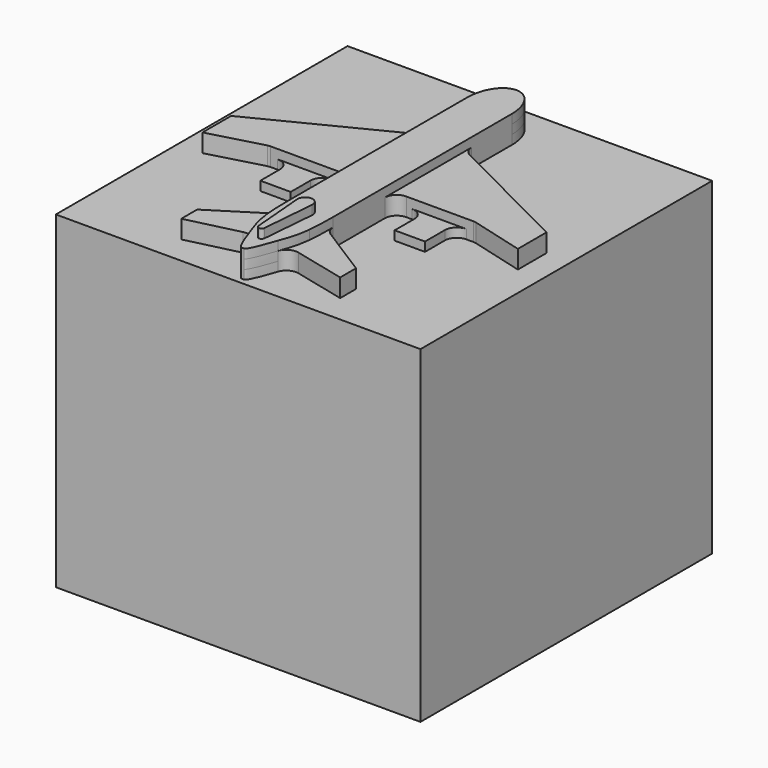
from build123d import *

# Parameters (mm, degrees)
F0_W     = 200
F0_H     = 200
F1_DEPTH = 180
F2_DEPTH = 185
F3_DEPTH = 190
F4_DEPTH = 195
F6_DEPTH = 5


with BuildPart() as f1:
    # F0 (on Top) → F1 (new body)
    with BuildSketch(Plane.XY):
        with Locations((0, -3.2757742546)):
            Rectangle(F0_W, F0_H)
        with BuildLine():
            Line((-12.2293280438, 41.5102764964), (-12.2293280438, 69.0648630261))
            add(Edge.make_bspline(
                [(12.2293280438, 69.0648630261), (12.2293280438, 87.5228339701), (0, 87.5228339701), (-12.2293280438, 87.5228339701), (-12.2293280438, 69.0648630261)],
                knots=[4.7123889804, 4.7123889804, 4.7123889804, 6.2831853072, 6.2831853072, 7.853981634, 7.853981634, 7.853981634], degree=2, weights=[1, 0.7071067812, 1, 0.7071067812, 1]))
            Line((12.2293280438, 69.0648630261), (12.2293280438, 41.5102764964))
            ThreePointArc((12.2293280438, 41.5102764964), (13.2009316357, 38.0774943136), (15.8274940025, 35.663125413))
            Line((15.8274940025, 35.663125413), (86.4709243178, 0))
            Line((86.4709243178, 0), (86.4709243178, -19.5954491359))
            Line((86.4709243178, -19.5954491359), (57.2512093193, -11.7076470548))
            ThreePointArc((57.2512093193, -11.7076470548), (56.4309868977, -11.5433023433), (55.5962785892, -11.488202028))
            Line((55.5962785892, -11.488202028), (51.7115545899, -11.488202028))
            ThreePointArc((51.7115545899, -11.488202028), (47.0800051731, -13.4066526112), (45.1615545899, -18.038202028))
            Line((45.1615545899, -18.038202028), (45.1615545899, -31.6096479073))
            Line((45.1615545899, -31.6096479073), (28.4984987229, -31.6096479073))
            Line((28.4984987229, -31.6096479073), (28.4984987229, -18.038202028))
            ThreePointArc((28.4984987229, -18.038202028), (26.5800481397, -13.4066526112), (21.9484987229, -11.488202028))
            Line((21.9484987229, -11.488202028), (18.7793280438, -11.488202028))
            ThreePointArc((18.7793280438, -11.488202028), (14.147778627, -13.4066526112), (12.2293280438, -18.038202028))
            Line((12.2293280438, -18.038202028), (12.2293280438, -53.4844789492))
            ThreePointArc((12.2293280438, -53.4844789492), (13.0425299585, -56.6454357234), (15.2802128465, -59.021508192))
            Line((15.2802128465, -59.021508192), (43.5760462728, -76.9030068116))
            Line((43.5760462728, -76.9030068116), (43.5760462728, -87.8098822028))
            Line((43.5760462728, -87.8098822028), (15.2160916988, -80.9541576008))
            ThreePointArc((15.2160916988, -80.9541576008), (10.5122070483, -81.586105591), (7.4700069214, -85.2290312635))
            add(Edge.make_bspline(
                [(7.4700069214, -85.2290312635), (4.8586251491, -93.3025441016), (1.9109145584, -100.0715989333), (0.7429708137, -100.072657045)],
                knots=[18.919621024, 18.919621024, 18.919621024, 18.919621024, 38.6142417327, 38.6142417327, 38.6142417327, 38.6142417327], degree=3))
            Line((0.7429708137, -100.072657045), (-0.7429708137, -100.072657045))
            add(Edge.make_bspline(
                [(-7.4700069214, -85.2290312635), (-4.8598522038, -93.3277695684), (-1.9207527988, -100.072657045), (-0.7429708137, -100.072657045)],
                knots=[19.243014526, 19.243014526, 19.243014526, 19.243014526, 39.0583236228, 39.0583236228, 39.0583236228, 39.0583236228], degree=3))
            ThreePointArc((-7.4700069214, -85.2290312635), (-10.5122070483, -81.586105591), (-15.2160916988, -80.9541576008))
            Line((-15.2160916988, -80.9541576008), (-43.5760462728, -87.8098822028))
            Line((-43.5760462728, -87.8098822028), (-43.5760462728, -76.9030068116))
            Line((-43.5760462728, -76.9030068116), (-15.2802128465, -59.021508192))
            ThreePointArc((-15.2802128465, -59.021508192), (-13.0425299585, -56.6454357234), (-12.2293280438, -53.4844789492))
            Line((-12.2293280438, -53.4844789492), (-12.2293280438, -18.038202028))
            ThreePointArc((-12.2293280438, -18.038202028), (-14.147778627, -13.4066526112), (-18.7793280438, -11.488202028))
            Line((-18.7793280438, -11.488202028), (-21.9484987229, -11.488202028))
            ThreePointArc((-21.9484987229, -11.488202028), (-26.5800481397, -13.4066526112), (-28.4984987229, -18.038202028))
            Line((-28.4984987229, -18.038202028), (-28.4984987229, -31.6096479073))
            Line((-28.4984987229, -31.6096479073), (-45.1615545899, -31.6096479073))
            Line((-45.1615545899, -31.6096479073), (-45.1615545899, -18.038202028))
            ThreePointArc((-45.1615545899, -18.038202028), (-47.0800051731, -13.4066526112), (-51.7115545899, -11.488202028))
            Line((-51.7115545899, -11.488202028), (-55.5962785892, -11.488202028))
            ThreePointArc((-55.5962785892, -11.488202028), (-56.4309868977, -11.5433023433), (-57.2512093193, -11.7076470548))
            Line((-57.2512093193, -11.7076470548), (-86.4709243178, -19.5954491359))
            Line((-86.4709243178, -19.5954491359), (-86.4709243178, 0))
            Line((-86.4709243178, 0), (-15.8274940025, 35.663125413))
            ThreePointArc((-15.8274940025, 35.663125413), (-13.2009316357, 38.0774943136), (-12.2293280438, 41.5102764964))
        make_face(mode=Mode.SUBTRACT)
        with BuildLine():
            add(Edge.make_bspline(
                [(12.2293280438, 69.0648630261), (12.2293280438, 87.5228339701), (0, 87.5228339701), (-12.2293280438, 87.5228339701), (-12.2293280438, 69.0648630261)],
                knots=[4.7123889804, 4.7123889804, 4.7123889804, 6.2831853072, 6.2831853072, 7.853981634, 7.853981634, 7.853981634], degree=2, weights=[1, 0.7071067812, 1, 0.7071067812, 1]))
            Line((-12.2293280438, 69.0648630261), (-12.2293280438, 41.5102764964))
            Line((-12.2293280438, 41.5102764964), (-12.2293280438, -18.038202028))
            Line((-12.2293280438, -18.038202028), (-12.2293280438, -53.4844789492))
            add(Edge.make_bspline(
                [(-12.2293280438, -53.4844789492), (-12.2293280438, -60.1853438847), (-12.0247001895, -64.9920828572), (-11.648149487, -68.7280764558)],
                knots=[0, 0, 0, 0, 10.5529945854, 10.5529945854, 10.5529945854, 10.5529945854], degree=3))
            add(Edge.make_bspline(
                [(-11.648149487, -68.7280764558), (-10.8243499192, -73.7523986697), (-9.2212130514, -79.7954222637), (-7.4700069214, -85.2290312635)],
                knots=[5.9485187923, 5.9485187923, 5.9485187923, 5.9485187923, 19.243014526, 19.243014526, 19.243014526, 19.243014526], degree=3))
            add(Edge.make_bspline(
                [(-7.4700069214, -85.2290312635), (-4.8598522038, -93.3277695684), (-1.9207527988, -100.072657045), (-0.7429708137, -100.072657045)],
                knots=[19.243014526, 19.243014526, 19.243014526, 19.243014526, 39.0583236228, 39.0583236228, 39.0583236228, 39.0583236228], degree=3))
            Line((-0.7429708137, -100.072657045), (0.7429708137, -100.072657045))
            add(Edge.make_bspline(
                [(7.4700069214, -85.2290312635), (4.8586251491, -93.3025441016), (1.9109145584, -100.0715989333), (0.7429708137, -100.072657045)],
                knots=[18.919621024, 18.919621024, 18.919621024, 18.919621024, 38.6142417327, 38.6142417327, 38.6142417327, 38.6142417327], degree=3))
            add(Edge.make_bspline(
                [(11.6358566621, -68.8490659918), (10.8266427242, -73.7935871479), (9.2242092605, -79.8056285057), (7.4700069214, -85.2290312635)],
                knots=[5.6897095333, 5.6897095333, 5.6897095333, 5.6897095333, 18.919621024, 18.919621024, 18.919621024, 18.919621024], degree=3))
            add(Edge.make_bspline(
                [(12.2293280438, -53.4844789492), (12.2293280438, -60.2579039154), (12.0202445878, -65.0959598972), (11.6358566621, -68.8490659918)],
                knots=[0, 0, 0, 0, 10.667267238, 10.667267238, 10.667267238, 10.667267238], degree=3))
            Line((12.2293280438, -53.4844789492), (12.2293280438, -18.038202028))
            Line((12.2293280438, -18.038202028), (12.2293280438, 41.5102764964))
            Line((12.2293280438, 41.5102764964), (12.2293280438, 69.0648630261))
        make_face()
        with BuildLine():
            Line((-12.2293280438, -18.038202028), (-12.2293280438, 41.5102764964))
            ThreePointArc((-12.2293280438, 41.5102764964), (-13.2009316357, 38.0774943136), (-15.8274940025, 35.663125413))
            Line((-15.8274940025, 35.663125413), (-86.4709243178, 0))
            Line((-86.4709243178, 0), (-86.4709243178, -19.5954491359))
            Line((-86.4709243178, -19.5954491359), (-57.2512093193, -11.7076470548))
            ThreePointArc((-57.2512093193, -11.7076470548), (-56.4309868977, -11.5433023433), (-55.5962785892, -11.488202028))
            Line((-55.5962785892, -11.488202028), (-51.7115545899, -11.488202028))
            Line((-51.7115545899, -11.488202028), (-21.9484987229, -11.488202028))
            Line((-21.9484987229, -11.488202028), (-18.7793280438, -11.488202028))
            ThreePointArc((-18.7793280438, -11.488202028), (-14.147778627, -13.4066526112), (-12.2293280438, -18.038202028))
        make_face()
        with BuildLine():
            ThreePointArc((15.8274940025, 35.663125413), (13.2009316357, 38.0774943136), (12.2293280438, 41.5102764964))
            Line((12.2293280438, 41.5102764964), (12.2293280438, -18.038202028))
            ThreePointArc((12.2293280438, -18.038202028), (14.147778627, -13.4066526112), (18.7793280438, -11.488202028))
            Line((18.7793280438, -11.488202028), (21.9484987229, -11.488202028))
            Line((21.9484987229, -11.488202028), (51.7115545899, -11.488202028))
            Line((51.7115545899, -11.488202028), (55.5962785892, -11.488202028))
            ThreePointArc((55.5962785892, -11.488202028), (56.4309868977, -11.5433023433), (57.2512093193, -11.7076470548))
            Line((57.2512093193, -11.7076470548), (86.4709243178, -19.5954491359))
            Line((86.4709243178, -19.5954491359), (86.4709243178, 0))
            Line((86.4709243178, 0), (15.8274940025, 35.663125413))
        make_face()
        with BuildLine():
            add(Edge.make_bspline(
                [(-12.2293280438, -53.4844789492), (-12.2293280438, -60.1853438847), (-12.0247001895, -64.9920828572), (-11.648149487, -68.7280764558)],
                knots=[0, 0, 0, 0, 10.5529945854, 10.5529945854, 10.5529945854, 10.5529945854], degree=3))
            ThreePointArc((-12.2293280438, -53.4844789492), (-13.0425299585, -56.6454357234), (-15.2802128465, -59.021508192))
            Line((-15.2802128465, -59.021508192), (-43.5760462728, -76.9030068116))
            Line((-43.5760462728, -76.9030068116), (-43.5760462728, -87.8098822028))
            Line((-43.5760462728, -87.8098822028), (-15.2160916988, -80.9541576008))
            ThreePointArc((-15.2160916988, -80.9541576008), (-10.5122070483, -81.586105591), (-7.4700069214, -85.2290312635))
            add(Edge.make_bspline(
                [(-11.648149487, -68.7280764558), (-10.8793352812, -76.3559601182), (-9.3938341658, -79.5202765414), (-7.4700069214, -85.2290312635)],
                knots=[10.5529945854, 10.5529945854, 10.5529945854, 10.5529945854, 32.0993417251, 32.0993417251, 32.0993417251, 32.0993417251], degree=3))
        make_face()
        with BuildLine():
            add(Edge.make_bspline(
                [(-11.648149487, -68.7280764558), (-10.8243499192, -73.7523986697), (-9.2212130514, -79.7954222637), (-7.4700069214, -85.2290312635)],
                knots=[5.9485187923, 5.9485187923, 5.9485187923, 5.9485187923, 19.243014526, 19.243014526, 19.243014526, 19.243014526], degree=3))
            add(Edge.make_bspline(
                [(-11.648149487, -68.7280764558), (-10.8793352812, -76.3559601182), (-9.3938341658, -79.5202765414), (-7.4700069214, -85.2290312635)],
                knots=[10.5529945854, 10.5529945854, 10.5529945854, 10.5529945854, 32.0993417251, 32.0993417251, 32.0993417251, 32.0993417251], degree=3))
        make_face()
        with BuildLine():
            ThreePointArc((-28.4984987229, -18.038202028), (-26.5800481397, -13.4066526112), (-21.9484987229, -11.488202028))
            Line((-21.9484987229, -11.488202028), (-51.7115545899, -11.488202028))
            ThreePointArc((-51.7115545899, -11.488202028), (-47.0800051731, -13.4066526112), (-45.1615545899, -18.038202028))
            Line((-45.1615545899, -18.038202028), (-45.1615545899, -31.6096479073))
            Line((-45.1615545899, -31.6096479073), (-28.4984987229, -31.6096479073))
            Line((-28.4984987229, -31.6096479073), (-28.4984987229, -18.038202028))
        make_face()
        with BuildLine():
            ThreePointArc((15.2802128465, -59.021508192), (13.0425299585, -56.6454357234), (12.2293280438, -53.4844789492))
            add(Edge.make_bspline(
                [(12.2293280438, -53.4844789492), (12.2293280438, -60.2579039154), (12.0202445878, -65.0959598972), (11.6358566621, -68.8490659918)],
                knots=[0, 0, 0, 0, 10.667267238, 10.667267238, 10.667267238, 10.667267238], degree=3))
            add(Edge.make_bspline(
                [(11.6358566621, -68.8490659918), (10.863566021, -76.3895960623), (9.3836310051, -79.5505533461), (7.4700069214, -85.2290312635)],
                knots=[10.667267238, 10.667267238, 10.667267238, 10.667267238, 32.0993417251, 32.0993417251, 32.0993417251, 32.0993417251], degree=3))
            ThreePointArc((7.4700069214, -85.2290312635), (10.5122070483, -81.586105591), (15.2160916988, -80.9541576008))
            Line((15.2160916988, -80.9541576008), (43.5760462728, -87.8098822028))
            Line((43.5760462728, -87.8098822028), (43.5760462728, -76.9030068116))
            Line((43.5760462728, -76.9030068116), (15.2802128465, -59.021508192))
        make_face()
        with BuildLine():
            Line((51.7115545899, -11.488202028), (21.9484987229, -11.488202028))
            ThreePointArc((21.9484987229, -11.488202028), (26.5800481397, -13.4066526112), (28.4984987229, -18.038202028))
            Line((28.4984987229, -18.038202028), (28.4984987229, -31.6096479073))
            Line((28.4984987229, -31.6096479073), (45.1615545899, -31.6096479073))
            Line((45.1615545899, -31.6096479073), (45.1615545899, -18.038202028))
            ThreePointArc((45.1615545899, -18.038202028), (47.0800051731, -13.4066526112), (51.7115545899, -11.488202028))
        make_face()
        with BuildLine():
            add(Edge.make_bspline(
                [(11.6358566621, -68.8490659918), (10.863566021, -76.3895960623), (9.3836310051, -79.5505533461), (7.4700069214, -85.2290312635)],
                knots=[10.667267238, 10.667267238, 10.667267238, 10.667267238, 32.0993417251, 32.0993417251, 32.0993417251, 32.0993417251], degree=3))
            add(Edge.make_bspline(
                [(11.6358566621, -68.8490659918), (10.8266427242, -73.7935871479), (9.2242092605, -79.8056285057), (7.4700069214, -85.2290312635)],
                knots=[5.6897095333, 5.6897095333, 5.6897095333, 5.6897095333, 18.919621024, 18.919621024, 18.919621024, 18.919621024], degree=3))
        make_face()
    extrude(amount=F1_DEPTH)

    # F0 (on Top) → F2 (join)
    with BuildSketch(Plane.XY):
        with BuildLine():
            Line((-12.2293280438, -18.038202028), (-12.2293280438, 41.5102764964))
            ThreePointArc((-12.2293280438, 41.5102764964), (-13.2009316357, 38.0774943136), (-15.8274940025, 35.663125413))
            Line((-15.8274940025, 35.663125413), (-86.4709243178, 0))
            Line((-86.4709243178, 0), (-86.4709243178, -19.5954491359))
            Line((-86.4709243178, -19.5954491359), (-57.2512093193, -11.7076470548))
            ThreePointArc((-57.2512093193, -11.7076470548), (-56.4309868977, -11.5433023433), (-55.5962785892, -11.488202028))
            Line((-55.5962785892, -11.488202028), (-51.7115545899, -11.488202028))
            Line((-51.7115545899, -11.488202028), (-21.9484987229, -11.488202028))
            Line((-21.9484987229, -11.488202028), (-18.7793280438, -11.488202028))
            ThreePointArc((-18.7793280438, -11.488202028), (-14.147778627, -13.4066526112), (-12.2293280438, -18.038202028))
        make_face()
        with BuildLine():
            ThreePointArc((-28.4984987229, -18.038202028), (-26.5800481397, -13.4066526112), (-21.9484987229, -11.488202028))
            Line((-21.9484987229, -11.488202028), (-51.7115545899, -11.488202028))
            ThreePointArc((-51.7115545899, -11.488202028), (-47.0800051731, -13.4066526112), (-45.1615545899, -18.038202028))
            Line((-45.1615545899, -18.038202028), (-45.1615545899, -31.6096479073))
            Line((-45.1615545899, -31.6096479073), (-28.4984987229, -31.6096479073))
            Line((-28.4984987229, -31.6096479073), (-28.4984987229, -18.038202028))
        make_face()
        with BuildLine():
            add(Edge.make_bspline(
                [(12.2293280438, 69.0648630261), (12.2293280438, 87.5228339701), (0, 87.5228339701), (-12.2293280438, 87.5228339701), (-12.2293280438, 69.0648630261)],
                knots=[4.7123889804, 4.7123889804, 4.7123889804, 6.2831853072, 6.2831853072, 7.853981634, 7.853981634, 7.853981634], degree=2, weights=[1, 0.7071067812, 1, 0.7071067812, 1]))
            Line((-12.2293280438, 69.0648630261), (-12.2293280438, 41.5102764964))
            Line((-12.2293280438, 41.5102764964), (-12.2293280438, -18.038202028))
            Line((-12.2293280438, -18.038202028), (-12.2293280438, -53.4844789492))
            add(Edge.make_bspline(
                [(-12.2293280438, -53.4844789492), (-12.2293280438, -60.1853438847), (-12.0247001895, -64.9920828572), (-11.648149487, -68.7280764558)],
                knots=[0, 0, 0, 0, 10.5529945854, 10.5529945854, 10.5529945854, 10.5529945854], degree=3))
            add(Edge.make_bspline(
                [(-11.648149487, -68.7280764558), (-10.8243499192, -73.7523986697), (-9.2212130514, -79.7954222637), (-7.4700069214, -85.2290312635)],
                knots=[5.9485187923, 5.9485187923, 5.9485187923, 5.9485187923, 19.243014526, 19.243014526, 19.243014526, 19.243014526], degree=3))
            add(Edge.make_bspline(
                [(-7.4700069214, -85.2290312635), (-4.8598522038, -93.3277695684), (-1.9207527988, -100.072657045), (-0.7429708137, -100.072657045)],
                knots=[19.243014526, 19.243014526, 19.243014526, 19.243014526, 39.0583236228, 39.0583236228, 39.0583236228, 39.0583236228], degree=3))
            Line((-0.7429708137, -100.072657045), (0.7429708137, -100.072657045))
            add(Edge.make_bspline(
                [(7.4700069214, -85.2290312635), (4.8586251491, -93.3025441016), (1.9109145584, -100.0715989333), (0.7429708137, -100.072657045)],
                knots=[18.919621024, 18.919621024, 18.919621024, 18.919621024, 38.6142417327, 38.6142417327, 38.6142417327, 38.6142417327], degree=3))
            add(Edge.make_bspline(
                [(11.6358566621, -68.8490659918), (10.8266427242, -73.7935871479), (9.2242092605, -79.8056285057), (7.4700069214, -85.2290312635)],
                knots=[5.6897095333, 5.6897095333, 5.6897095333, 5.6897095333, 18.919621024, 18.919621024, 18.919621024, 18.919621024], degree=3))
            add(Edge.make_bspline(
                [(12.2293280438, -53.4844789492), (12.2293280438, -60.2579039154), (12.0202445878, -65.0959598972), (11.6358566621, -68.8490659918)],
                knots=[0, 0, 0, 0, 10.667267238, 10.667267238, 10.667267238, 10.667267238], degree=3))
            Line((12.2293280438, -53.4844789492), (12.2293280438, -18.038202028))
            Line((12.2293280438, -18.038202028), (12.2293280438, 41.5102764964))
            Line((12.2293280438, 41.5102764964), (12.2293280438, 69.0648630261))
        make_face()
        with BuildLine():
            ThreePointArc((15.8274940025, 35.663125413), (13.2009316357, 38.0774943136), (12.2293280438, 41.5102764964))
            Line((12.2293280438, 41.5102764964), (12.2293280438, -18.038202028))
            ThreePointArc((12.2293280438, -18.038202028), (14.147778627, -13.4066526112), (18.7793280438, -11.488202028))
            Line((18.7793280438, -11.488202028), (21.9484987229, -11.488202028))
            Line((21.9484987229, -11.488202028), (51.7115545899, -11.488202028))
            Line((51.7115545899, -11.488202028), (55.5962785892, -11.488202028))
            ThreePointArc((55.5962785892, -11.488202028), (56.4309868977, -11.5433023433), (57.2512093193, -11.7076470548))
            Line((57.2512093193, -11.7076470548), (86.4709243178, -19.5954491359))
            Line((86.4709243178, -19.5954491359), (86.4709243178, 0))
            Line((86.4709243178, 0), (15.8274940025, 35.663125413))
        make_face()
        with BuildLine():
            Line((51.7115545899, -11.488202028), (21.9484987229, -11.488202028))
            ThreePointArc((21.9484987229, -11.488202028), (26.5800481397, -13.4066526112), (28.4984987229, -18.038202028))
            Line((28.4984987229, -18.038202028), (28.4984987229, -31.6096479073))
            Line((28.4984987229, -31.6096479073), (45.1615545899, -31.6096479073))
            Line((45.1615545899, -31.6096479073), (45.1615545899, -18.038202028))
            ThreePointArc((45.1615545899, -18.038202028), (47.0800051731, -13.4066526112), (51.7115545899, -11.488202028))
        make_face()
        with BuildLine():
            ThreePointArc((15.2802128465, -59.021508192), (13.0425299585, -56.6454357234), (12.2293280438, -53.4844789492))
            add(Edge.make_bspline(
                [(12.2293280438, -53.4844789492), (12.2293280438, -60.2579039154), (12.0202445878, -65.0959598972), (11.6358566621, -68.8490659918)],
                knots=[0, 0, 0, 0, 10.667267238, 10.667267238, 10.667267238, 10.667267238], degree=3))
            add(Edge.make_bspline(
                [(11.6358566621, -68.8490659918), (10.863566021, -76.3895960623), (9.3836310051, -79.5505533461), (7.4700069214, -85.2290312635)],
                knots=[10.667267238, 10.667267238, 10.667267238, 10.667267238, 32.0993417251, 32.0993417251, 32.0993417251, 32.0993417251], degree=3))
            ThreePointArc((7.4700069214, -85.2290312635), (10.5122070483, -81.586105591), (15.2160916988, -80.9541576008))
            Line((15.2160916988, -80.9541576008), (43.5760462728, -87.8098822028))
            Line((43.5760462728, -87.8098822028), (43.5760462728, -76.9030068116))
            Line((43.5760462728, -76.9030068116), (15.2802128465, -59.021508192))
        make_face()
        with BuildLine():
            add(Edge.make_bspline(
                [(-12.2293280438, -53.4844789492), (-12.2293280438, -60.1853438847), (-12.0247001895, -64.9920828572), (-11.648149487, -68.7280764558)],
                knots=[0, 0, 0, 0, 10.5529945854, 10.5529945854, 10.5529945854, 10.5529945854], degree=3))
            ThreePointArc((-12.2293280438, -53.4844789492), (-13.0425299585, -56.6454357234), (-15.2802128465, -59.021508192))
            Line((-15.2802128465, -59.021508192), (-43.5760462728, -76.9030068116))
            Line((-43.5760462728, -76.9030068116), (-43.5760462728, -87.8098822028))
            Line((-43.5760462728, -87.8098822028), (-15.2160916988, -80.9541576008))
            ThreePointArc((-15.2160916988, -80.9541576008), (-10.5122070483, -81.586105591), (-7.4700069214, -85.2290312635))
            add(Edge.make_bspline(
                [(-11.648149487, -68.7280764558), (-10.8793352812, -76.3559601182), (-9.3938341658, -79.5202765414), (-7.4700069214, -85.2290312635)],
                knots=[10.5529945854, 10.5529945854, 10.5529945854, 10.5529945854, 32.0993417251, 32.0993417251, 32.0993417251, 32.0993417251], degree=3))
        make_face()
    extrude(amount=F2_DEPTH)

    # F0 (on Top) → F3 (join)
    with BuildSketch(Plane.XY):
        with BuildLine():
            add(Edge.make_bspline(
                [(12.2293280438, 69.0648630261), (12.2293280438, 87.5228339701), (0, 87.5228339701), (-12.2293280438, 87.5228339701), (-12.2293280438, 69.0648630261)],
                knots=[4.7123889804, 4.7123889804, 4.7123889804, 6.2831853072, 6.2831853072, 7.853981634, 7.853981634, 7.853981634], degree=2, weights=[1, 0.7071067812, 1, 0.7071067812, 1]))
            Line((-12.2293280438, 69.0648630261), (-12.2293280438, 41.5102764964))
            Line((-12.2293280438, 41.5102764964), (-12.2293280438, -18.038202028))
            Line((-12.2293280438, -18.038202028), (-12.2293280438, -53.4844789492))
            add(Edge.make_bspline(
                [(-12.2293280438, -53.4844789492), (-12.2293280438, -60.1853438847), (-12.0247001895, -64.9920828572), (-11.648149487, -68.7280764558)],
                knots=[0, 0, 0, 0, 10.5529945854, 10.5529945854, 10.5529945854, 10.5529945854], degree=3))
            add(Edge.make_bspline(
                [(-11.648149487, -68.7280764558), (-10.8243499192, -73.7523986697), (-9.2212130514, -79.7954222637), (-7.4700069214, -85.2290312635)],
                knots=[5.9485187923, 5.9485187923, 5.9485187923, 5.9485187923, 19.243014526, 19.243014526, 19.243014526, 19.243014526], degree=3))
            add(Edge.make_bspline(
                [(-7.4700069214, -85.2290312635), (-4.8598522038, -93.3277695684), (-1.9207527988, -100.072657045), (-0.7429708137, -100.072657045)],
                knots=[19.243014526, 19.243014526, 19.243014526, 19.243014526, 39.0583236228, 39.0583236228, 39.0583236228, 39.0583236228], degree=3))
            Line((-0.7429708137, -100.072657045), (0.7429708137, -100.072657045))
            add(Edge.make_bspline(
                [(7.4700069214, -85.2290312635), (4.8586251491, -93.3025441016), (1.9109145584, -100.0715989333), (0.7429708137, -100.072657045)],
                knots=[18.919621024, 18.919621024, 18.919621024, 18.919621024, 38.6142417327, 38.6142417327, 38.6142417327, 38.6142417327], degree=3))
            add(Edge.make_bspline(
                [(11.6358566621, -68.8490659918), (10.8266427242, -73.7935871479), (9.2242092605, -79.8056285057), (7.4700069214, -85.2290312635)],
                knots=[5.6897095333, 5.6897095333, 5.6897095333, 5.6897095333, 18.919621024, 18.919621024, 18.919621024, 18.919621024], degree=3))
            add(Edge.make_bspline(
                [(12.2293280438, -53.4844789492), (12.2293280438, -60.2579039154), (12.0202445878, -65.0959598972), (11.6358566621, -68.8490659918)],
                knots=[0, 0, 0, 0, 10.667267238, 10.667267238, 10.667267238, 10.667267238], degree=3))
            Line((12.2293280438, -53.4844789492), (12.2293280438, -18.038202028))
            Line((12.2293280438, -18.038202028), (12.2293280438, 41.5102764964))
            Line((12.2293280438, 41.5102764964), (12.2293280438, 69.0648630261))
        make_face()
        with BuildLine():
            Line((-12.2293280438, -18.038202028), (-12.2293280438, 41.5102764964))
            ThreePointArc((-12.2293280438, 41.5102764964), (-13.2009316357, 38.0774943136), (-15.8274940025, 35.663125413))
            Line((-15.8274940025, 35.663125413), (-86.4709243178, 0))
            Line((-86.4709243178, 0), (-86.4709243178, -19.5954491359))
            Line((-86.4709243178, -19.5954491359), (-57.2512093193, -11.7076470548))
            ThreePointArc((-57.2512093193, -11.7076470548), (-56.4309868977, -11.5433023433), (-55.5962785892, -11.488202028))
            Line((-55.5962785892, -11.488202028), (-51.7115545899, -11.488202028))
            Line((-51.7115545899, -11.488202028), (-21.9484987229, -11.488202028))
            Line((-21.9484987229, -11.488202028), (-18.7793280438, -11.488202028))
            ThreePointArc((-18.7793280438, -11.488202028), (-14.147778627, -13.4066526112), (-12.2293280438, -18.038202028))
        make_face()
        with BuildLine():
            ThreePointArc((15.8274940025, 35.663125413), (13.2009316357, 38.0774943136), (12.2293280438, 41.5102764964))
            Line((12.2293280438, 41.5102764964), (12.2293280438, -18.038202028))
            ThreePointArc((12.2293280438, -18.038202028), (14.147778627, -13.4066526112), (18.7793280438, -11.488202028))
            Line((18.7793280438, -11.488202028), (21.9484987229, -11.488202028))
            Line((21.9484987229, -11.488202028), (51.7115545899, -11.488202028))
            Line((51.7115545899, -11.488202028), (55.5962785892, -11.488202028))
            ThreePointArc((55.5962785892, -11.488202028), (56.4309868977, -11.5433023433), (57.2512093193, -11.7076470548))
            Line((57.2512093193, -11.7076470548), (86.4709243178, -19.5954491359))
            Line((86.4709243178, -19.5954491359), (86.4709243178, 0))
            Line((86.4709243178, 0), (15.8274940025, 35.663125413))
        make_face()
        with BuildLine():
            ThreePointArc((15.2802128465, -59.021508192), (13.0425299585, -56.6454357234), (12.2293280438, -53.4844789492))
            add(Edge.make_bspline(
                [(12.2293280438, -53.4844789492), (12.2293280438, -60.2579039154), (12.0202445878, -65.0959598972), (11.6358566621, -68.8490659918)],
                knots=[0, 0, 0, 0, 10.667267238, 10.667267238, 10.667267238, 10.667267238], degree=3))
            add(Edge.make_bspline(
                [(11.6358566621, -68.8490659918), (10.863566021, -76.3895960623), (9.3836310051, -79.5505533461), (7.4700069214, -85.2290312635)],
                knots=[10.667267238, 10.667267238, 10.667267238, 10.667267238, 32.0993417251, 32.0993417251, 32.0993417251, 32.0993417251], degree=3))
            ThreePointArc((7.4700069214, -85.2290312635), (10.5122070483, -81.586105591), (15.2160916988, -80.9541576008))
            Line((15.2160916988, -80.9541576008), (43.5760462728, -87.8098822028))
            Line((43.5760462728, -87.8098822028), (43.5760462728, -76.9030068116))
            Line((43.5760462728, -76.9030068116), (15.2802128465, -59.021508192))
        make_face()
        with BuildLine():
            add(Edge.make_bspline(
                [(-12.2293280438, -53.4844789492), (-12.2293280438, -60.1853438847), (-12.0247001895, -64.9920828572), (-11.648149487, -68.7280764558)],
                knots=[0, 0, 0, 0, 10.5529945854, 10.5529945854, 10.5529945854, 10.5529945854], degree=3))
            ThreePointArc((-12.2293280438, -53.4844789492), (-13.0425299585, -56.6454357234), (-15.2802128465, -59.021508192))
            Line((-15.2802128465, -59.021508192), (-43.5760462728, -76.9030068116))
            Line((-43.5760462728, -76.9030068116), (-43.5760462728, -87.8098822028))
            Line((-43.5760462728, -87.8098822028), (-15.2160916988, -80.9541576008))
            ThreePointArc((-15.2160916988, -80.9541576008), (-10.5122070483, -81.586105591), (-7.4700069214, -85.2290312635))
            add(Edge.make_bspline(
                [(-11.648149487, -68.7280764558), (-10.8793352812, -76.3559601182), (-9.3938341658, -79.5202765414), (-7.4700069214, -85.2290312635)],
                knots=[10.5529945854, 10.5529945854, 10.5529945854, 10.5529945854, 32.0993417251, 32.0993417251, 32.0993417251, 32.0993417251], degree=3))
        make_face()
    extrude(amount=F3_DEPTH)

    # F0 (on Top) → F4 (join)
    with BuildSketch(Plane.XY):
        with BuildLine():
            add(Edge.make_bspline(
                [(12.2293280438, 69.0648630261), (12.2293280438, 87.5228339701), (0, 87.5228339701), (-12.2293280438, 87.5228339701), (-12.2293280438, 69.0648630261)],
                knots=[4.7123889804, 4.7123889804, 4.7123889804, 6.2831853072, 6.2831853072, 7.853981634, 7.853981634, 7.853981634], degree=2, weights=[1, 0.7071067812, 1, 0.7071067812, 1]))
            Line((-12.2293280438, 69.0648630261), (-12.2293280438, 41.5102764964))
            Line((-12.2293280438, 41.5102764964), (-12.2293280438, -18.038202028))
            Line((-12.2293280438, -18.038202028), (-12.2293280438, -53.4844789492))
            add(Edge.make_bspline(
                [(-12.2293280438, -53.4844789492), (-12.2293280438, -60.1853438847), (-12.0247001895, -64.9920828572), (-11.648149487, -68.7280764558)],
                knots=[0, 0, 0, 0, 10.5529945854, 10.5529945854, 10.5529945854, 10.5529945854], degree=3))
            add(Edge.make_bspline(
                [(-11.648149487, -68.7280764558), (-10.8243499192, -73.7523986697), (-9.2212130514, -79.7954222637), (-7.4700069214, -85.2290312635)],
                knots=[5.9485187923, 5.9485187923, 5.9485187923, 5.9485187923, 19.243014526, 19.243014526, 19.243014526, 19.243014526], degree=3))
            add(Edge.make_bspline(
                [(-7.4700069214, -85.2290312635), (-4.8598522038, -93.3277695684), (-1.9207527988, -100.072657045), (-0.7429708137, -100.072657045)],
                knots=[19.243014526, 19.243014526, 19.243014526, 19.243014526, 39.0583236228, 39.0583236228, 39.0583236228, 39.0583236228], degree=3))
            Line((-0.7429708137, -100.072657045), (0.7429708137, -100.072657045))
            add(Edge.make_bspline(
                [(7.4700069214, -85.2290312635), (4.8586251491, -93.3025441016), (1.9109145584, -100.0715989333), (0.7429708137, -100.072657045)],
                knots=[18.919621024, 18.919621024, 18.919621024, 18.919621024, 38.6142417327, 38.6142417327, 38.6142417327, 38.6142417327], degree=3))
            add(Edge.make_bspline(
                [(11.6358566621, -68.8490659918), (10.8266427242, -73.7935871479), (9.2242092605, -79.8056285057), (7.4700069214, -85.2290312635)],
                knots=[5.6897095333, 5.6897095333, 5.6897095333, 5.6897095333, 18.919621024, 18.919621024, 18.919621024, 18.919621024], degree=3))
            add(Edge.make_bspline(
                [(12.2293280438, -53.4844789492), (12.2293280438, -60.2579039154), (12.0202445878, -65.0959598972), (11.6358566621, -68.8490659918)],
                knots=[0, 0, 0, 0, 10.667267238, 10.667267238, 10.667267238, 10.667267238], degree=3))
            Line((12.2293280438, -53.4844789492), (12.2293280438, -18.038202028))
            Line((12.2293280438, -18.038202028), (12.2293280438, 41.5102764964))
            Line((12.2293280438, 41.5102764964), (12.2293280438, 69.0648630261))
        make_face()
        with BuildLine():
            add(Edge.make_bspline(
                [(-11.648149487, -68.7280764558), (-10.8243499192, -73.7523986697), (-9.2212130514, -79.7954222637), (-7.4700069214, -85.2290312635)],
                knots=[5.9485187923, 5.9485187923, 5.9485187923, 5.9485187923, 19.243014526, 19.243014526, 19.243014526, 19.243014526], degree=3))
            add(Edge.make_bspline(
                [(-11.648149487, -68.7280764558), (-10.8793352812, -76.3559601182), (-9.3938341658, -79.5202765414), (-7.4700069214, -85.2290312635)],
                knots=[10.5529945854, 10.5529945854, 10.5529945854, 10.5529945854, 32.0993417251, 32.0993417251, 32.0993417251, 32.0993417251], degree=3))
        make_face()
        with BuildLine():
            add(Edge.make_bspline(
                [(11.6358566621, -68.8490659918), (10.863566021, -76.3895960623), (9.3836310051, -79.5505533461), (7.4700069214, -85.2290312635)],
                knots=[10.667267238, 10.667267238, 10.667267238, 10.667267238, 32.0993417251, 32.0993417251, 32.0993417251, 32.0993417251], degree=3))
            add(Edge.make_bspline(
                [(11.6358566621, -68.8490659918), (10.8266427242, -73.7935871479), (9.2242092605, -79.8056285057), (7.4700069214, -85.2290312635)],
                knots=[5.6897095333, 5.6897095333, 5.6897095333, 5.6897095333, 18.919621024, 18.919621024, 18.919621024, 18.919621024], degree=3))
        make_face()
    extrude(amount=F4_DEPTH)

    # F5 (on face) → F6 (join)
    with BuildSketch(Plane.XY.offset(195)):
        with BuildLine():
            ThreePointArc((4.1187503375, -57.6947666705), (0, -53.2144096197), (-4.1187503375, -57.6947666705))
            Line((-4.1187503375, -57.6947666705), (-1.6269049374, -87.2707590461))
            ThreePointArc((-1.6269049374, -87.2707590461), (0, -88.7663575406), (1.6269049374, -87.2707590461))
            Line((1.6269049374, -87.2707590461), (4.1187503375, -57.6947666705))
        make_face()
    extrude(amount=F6_DEPTH)


solid = f1.part
